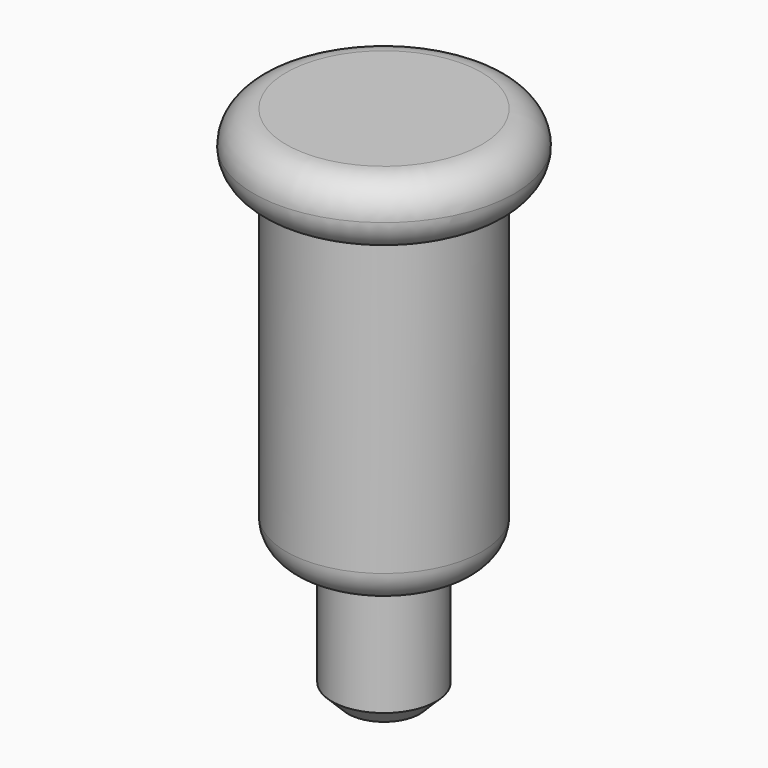
from build123d import *

# Parameters (mm, degrees)
F2_R     = 0.49999
F3_SIZE2 = 0.25
F3_SIZE  = 0.25


# Not quite as in the source:
# - a fillet or chamfer is up to 0.001 mm smaller than in the source, because OpenCascade refuses the exact size


with BuildPart() as f1:
    # F0 (on Front) → F1 (revolve)
    with BuildSketch(Plane.XZ):
        Polygon((0, 8), (0, 0), (0.8, 0), (0.8, 2), (1.5, 2), (1.5, 7), (2, 7), (2, 8), align=None)
    revolve(axis=Axis((0, 0, 4), (0, 0, 1)))

    # F2 (radius 0.5 in the source; OpenCascade refuses exactly that, so slightly less here)
    f2_edges = [f1.edges().sort_by_distance(p)[0] for p in [
        (-2, 0, 7),
        (-2, 0, 8),
        (2, 0, 7.5),
        (-1.5, 0, 2),
    ]]
    fillet(f2_edges, radius=F2_R)

    # F3
    f3_edges = [f1.edges().sort_by_distance(p)[0] for p in [
        (-0.8, 0, 0),
    ]]
    chamfer(f3_edges, length=F3_SIZE, length2=F3_SIZE2)


solid = f1.part
